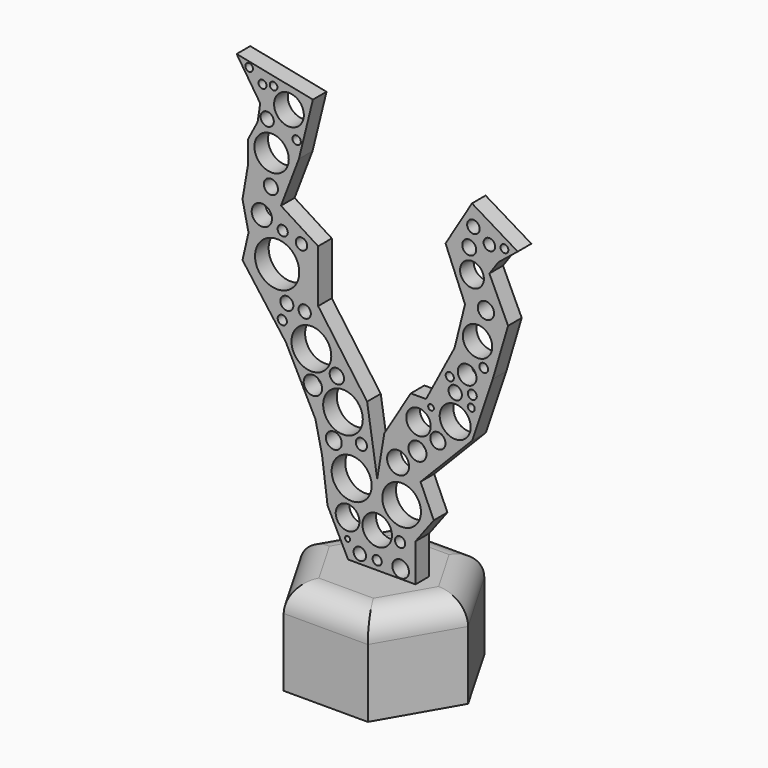
from build123d import *

# Parameters (mm, degrees)
F1_DEPTH = 22
F2_R     = 6
F3_W     = 66
F3_H     = 4
F4_DEPTH = 96
F5_R     = 4.6734146419
F5_R_2   = 4.6518685429
F5_R_3   = 4.696387476
F5_R_4   = 4.5347148874
F5_R_5   = 2.5803932982
F5_R_6   = 2.1193315606
F5_R_7   = 2.8799856964
F5_R_8   = 3.6433218135
F5_R_9   = 1.5618927534
F5_R_10  = 1.780828752
F5_R_11  = 1.3177092187
F5_R_12  = 1.8635222484
F5_R_13  = 1.68135752
F5_R_14  = 2.1595766427
F5_R_15  = 1.0781288147
F5_R_16  = 1.4474492092
F5_R_17  = 2.7862850737
F5_R_18  = 3.4582862602
F5_R_19  = 1.9500679084
F5_R_20  = 1.1979173869
F5_R_21  = 1.4573267426
F5_R_22  = 1.0781294395
F5_R_23  = 0.5989588797
F5_R_24  = 3.4929735647
F5_R_25  = 4.0355453194
F5_R_26  = 5.1927529479
F5_R_27  = 2.3790588204
F5_R_28  = 2.1982450571
F5_R_29  = 3.4468016913
F5_R_30  = 2.7968598425
F5_R_31  = 1.4614439331
F5_R_32  = 1.3473825629
F5_R_33  = 1.6339413822
F5_R_34  = 1.9124784447
F5_R_35  = 1.6663004851
F5_R_36  = 1.3473821111
F5_R_37  = 1.521199858
F5_R_38  = 1.189529666
F5_R_39  = 0.9803697467
F5_R_40  = 0.8958556794
F5_R_41  = 0.9362344169
F5_R_42  = 0.9000294175
F5_R_43  = 1.5546857265
F5_R_44  = 1.0528691723
F5_R_45  = 0.9573948707
F5_R_46  = 1.0252641854
F5_R_47  = 0.8253231645
F5_R_48  = 0.6675992995
F5_R_49  = 0.9215911414
F6_DEPTH = 19.0993858407


# Not quite as in the source:
# - a feature names something its author has since deleted; it is built from what else it names


with BuildPart() as f1:
    # F0 (on Top) → F1 (new body)
    with BuildSketch(Plane.XY):
        Polygon((9.8717576678, 17.0983858407), (-9.8717576678, 17.0983858407), (-19.7435153356, 0), (-9.8717576678, -17.0983858407), (9.8717576678, -17.0983858407), (19.7435153356, 0), align=None)
    extrude(amount=F1_DEPTH)

    # F2
    f2_edges = [f1.edges().sort_by_distance(p)[0] for p in [
        (14.807637, 8.549193, 22),
        (0, 17.098386, 22),
        (-14.807637, 8.549193, 22),
        (-14.807637, -8.549193, 22),
        (0, -17.098386, 22),
        (14.807637, -8.549193, 22),
    ]]
    fillet(f2_edges, radius=F2_R)

    # F3 (on face) → F4 (join)
    with BuildSketch(Plane.XY.offset(22)):
        Rectangle(F3_W, F3_H)
    extrude(amount=F4_DEPTH)

    # F5 (on face) → F6 (cut, through all)
    with BuildSketch(Plane.XZ.offset(2)):
        with Locations((-15.4567928985, 62.7651289105)):
            Circle(F5_R)
        with Locations((-8.0297058448, 52.103664726)):
            Circle(F5_R_2)
        with Locations((-5.9932461008, 39.0463657677)):
            Circle(F5_R_3)
        with Locations((5.7463436387, 37.3692810535)):
            Circle(F5_R_4)
        with Locations((4.9078003503, 45.8744950593)):
            Circle(F5_R_5)
        with Locations((9.4598866999, 49.7078299522)):
            Circle(F5_R_6)
        with Locations((9.6994703636, 55.8172091842)):
            Circle(F5_R_7)
        with Locations((18.3244738728, 58.6922094226)):
            Circle(F5_R_8)
        with Locations((18.3244738728, 64.6817982197)):
            Circle(F5_R_9)
        with Locations((14.2515562475, 53.4213744104)):
            Circle(F5_R_10)
        with Locations((-3.7172031589, 46.8328297138)):
            Circle(F5_R_11)
        with Locations((-10.185956955, 45.5151200294)):
            Circle(F5_R_12)
        with Locations((-9.467205964, 59.0515844524)):
            Circle(F5_R_13)
        with Locations((-15.0974178687, 55.3380399942)):
            Circle(F5_R_14)
        with Locations((-22.2849212587, 66.4786696434)):
            Circle(F5_R_15)
        with Locations((-17.0140843838, 69.9526295066)):
            Circle(F5_R_16)
        with Locations((-6.9515802898, 30.6609440595)):
            Circle(F5_R_17)
        with Locations((0, 30.3015690297)):
            Circle(F5_R_18)
        with Locations((5.5067595094, 24.0724012256)):
            Circle(F5_R_19)
        with Locations((5.3869681433, 29.5828189701)):
            Circle(F5_R_20)
        with Locations((-4.0765781887, 24.0724012256)):
            Circle(F5_R_21)
        with Locations((0, 24.0724012256)):
            Circle(F5_R_22)
        with Locations((-6.9515802898, 26.2286514044)):
            Circle(F5_R_23)
        with Locations((-20.7141488791, 110.4762628675)):
            Circle(F5_R_24)
        with Locations((-24.7990079224, 100.1824140549)):
            Circle(F5_R_25)
        with Locations((-23.4918538481, 77.6339918375)):
            Circle(F5_R_26)
        with Locations((-27.0865298808, 86.6206809878)):
            Circle(F5_R_27)
        with Locations((21.1148075759, 69.3008825183)):
            Circle(F5_R_28)
        with Locations((23.5657226294, 76.980419457)):
            Circle(F5_R_29)
        with Locations((22.2585685551, 90.3787538409)):
            Circle(F5_R_30)
        with Locations((22.585356608, 100.3458127379)):
            Circle(F5_R_31)
        with Locations((26.3434294611, 97.8948995471)):
            Circle(F5_R_32)
        with Locations((21.6049905866, 95.7707688212)):
            Circle(F5_R_33)
        with Locations((25.5264546722, 84.0063765645)):
            Circle(F5_R_34)
        with Locations((-24.9624028802, 93.1564569473)):
            Circle(F5_R_35)
        with Locations((-17.7730508149, 83.6795866489)):
            Circle(F5_R_36)
        with Locations((-21.2043337524, 70.2812448144)):
            Circle(F5_R_37)
        with Locations((-22.1846997738, 84.9867388606)):
            Circle(F5_R_38)
        with Locations((-18.916811794, 104.7574579716)):
            Circle(F5_R_39)
        with Locations((-30.0772096962, 116.170220077)):
            Circle(F5_R_40)
        with Locations((-26.9252173603, 113.7220710516)):
            Circle(F5_R_41)
        with Locations((-24.3240576237, 114.1811013222)):
            Circle(F5_R_42)
        with Locations((-25.8235502988, 106.8672537804)):
            Circle(F5_R_43)
        with Locations((22.332961016, 65.5509606004)):
            Circle(F5_R_44)
        with Locations((17.0422960073, 67.5684064627)):
            Circle(F5_R_45)
        with Locations((25.0203702599, 71.9701051712)):
            Circle(F5_R_46)
        with Locations((22.0859050751, 62.7999007702)):
            Circle(F5_R_47)
        with Locations((12.6406000927, 59.7737394273)):
            Circle(F5_R_48)
        with Locations((29.8805739731, 98.1968715787)):
            Circle(F5_R_49)
        Polygon((-11.660611567, 22), (-6.8317884579, 22), (-11.660611567, 31.6260260755), (-12.9401380399, 41.5687402004), (-14.4974304566, 48.5166599268), (-21.445350183, 62.1729185099), (-31.6276470402, 75.8291770929), (-30.214605853, 81.9581896067), (-31.6276470402, 88.4158834815), (-30.3520038724, 95.8353579044), (-30.3520038724, 101.1938676238), (-28.0701080944, 105.5646776068), (-27.4666510522, 109.5751300454), (-33, 118), (-33, 22), align=None)
        Polygon((33, 118), (-33, 118), (-15.0963891501, 114.3840551376), (-18.3763280511, 101.0725870728), (-22.5977953523, 90.0094285607), (-13.8637246564, 84.4778493047), (-13.8637246564, 72.1045807004), (-2.3638659623, 56.0921244323), (0, 40.8702604473), (1.6708788462, 50.837315619), (7.8798653558, 61.1311607063), (11.4745413885, 61.1311607063), (18.1737095118, 73.875926435), (20.6246245652, 83.6795866489), (16.0495843738, 94.7903990746), (22.2585685551, 105.0842478871), (33, 98.6052934028), align=None)
        Polygon((8.980720304, 30.9005267918), (8.980720304, 22), (11.660611567, 22), (33, 22), (33, 98.6052934028), (28.467554599, 94.9537977576), (26.3434294611, 91.9126495719), (30.7337772995, 82.5414285064), (27.1243248135, 70.3275278211), (22.332961016, 56.0962293618), (10.1786367595, 43.5984507203), (13.2932206616, 36.6505309939), align=None)
    extrude(amount=-F6_DEPTH, mode=Mode.SUBTRACT)


solid = f1.part
